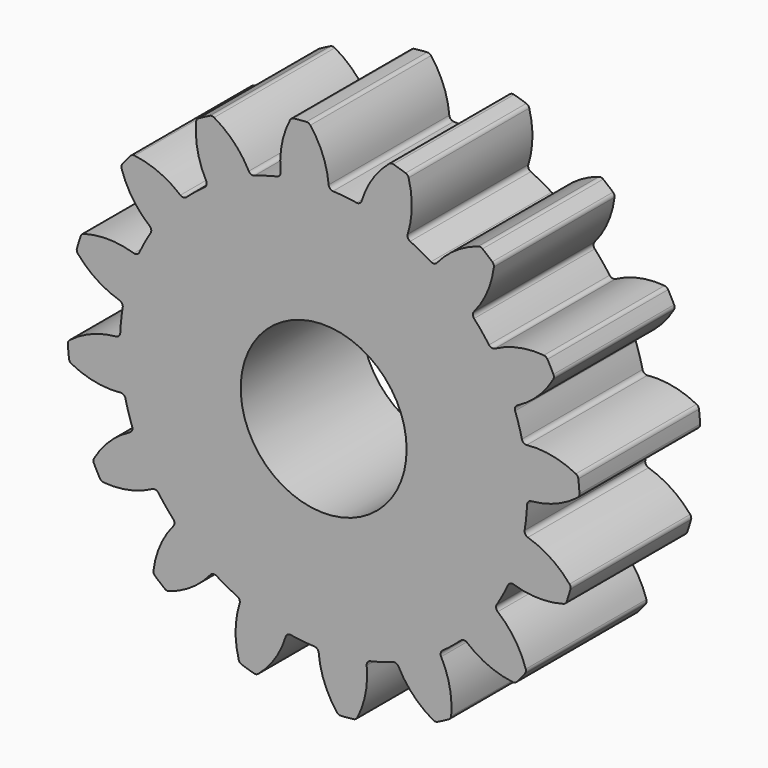
from build123d import *

# Parameters (mm, degrees)
F1_DEPTH = 2
F2_R     = 1.1
F3_DEPTH = 2.001


# Not quite as in the source:
# - a feature names something its author has since deleted; it is built from what else it names


with BuildPart() as f1:
    # F0 (on Front) → F1 (new body)
    with BuildSketch(Plane.XZ):
        with BuildLine():
            ThreePointArc((0.0658501888, 2.7527937353), (-0.0107962206, 3.0784970655), (-0.1768571825, 3.3689812963))
            ThreePointArc((-0.1768571825, 3.3689812963), (-0.2000460149, 3.3871150499), (-0.2290271151, 3.3922774917))
            ThreePointArc((-0.2290271151, 3.3922774917), (-0.3137124222, 3.3854961994), (-0.3982018601, 3.376601143))
            ThreePointArc((-0.3982018601, 3.376601143), (-0.4257409058, 3.3662013384), (-0.4452028358, 3.3441154096))
            ThreePointArc((-0.4452028358, 3.3441154096), (-0.5550599569, 3.0280636032), (-0.5705534857, 2.6938222503))
            ThreePointArc((-0.5705534857, 2.6938222503), (-0.5816569835, 2.6523658625), (-0.6173153418, 2.6284827884))
            ThreePointArc((-0.6173153418, 2.6284827884), (-0.7688345847, 2.5882220502), (-0.9177616204, 2.539234847))
            ThreePointArc((-0.9177616204, 2.539234847), (-1.258998717, 2.3884979026), (-1.5762018248, 2.1921650959))
            ThreePointArc((-1.5762018248, 2.1921650959), (-1.7007802346, 2.09698512), (-1.8196242836, 1.9947349364))
            ThreePointArc((-1.8196242836, 1.9947349364), (-2.0772017217, 1.7248863753), (-2.2951258682, 1.4221101396))
            ThreePointArc((-2.2951258682, 1.4221101396), (-2.3737975114, 1.2865012145), (-2.4444656446, 1.1465547141))
            ThreePointArc((-2.4444656446, 1.1465547141), (-2.5791695941, 0.7986765335), (-2.6646378036, 0.435551806))
            ThreePointArc((-2.6646378036, 0.435551806), (-2.6854256356, 0.2801591612), (-2.6971592704, 0.12382193))
            ThreePointArc((-2.6971592704, 0.12382193), (-2.688482276, -0.2491245706), (-2.6284827884, -0.6173153418))
            ThreePointArc((-2.6284827884, -0.6173153418), (-2.5882220502, -0.7688345847), (-2.539234847, -0.9177616204))
            ThreePointArc((-2.539234847, -0.9177616204), (-2.3884979026, -1.258998717), (-2.1921650959, -1.5762018248))
            ThreePointArc((-2.1921650959, -1.5762018248), (-2.09698512, -1.7007802346), (-1.9947349364, -1.8196242836))
            ThreePointArc((-1.9947349364, -1.8196242836), (-1.7248863753, -2.0772017217), (-1.4221101396, -2.2951258682))
            ThreePointArc((-1.4221101396, -2.2951258682), (-1.2865012145, -2.3737975114), (-1.1465547141, -2.4444656446))
            ThreePointArc((-1.1465547141, -2.4444656446), (-0.7986765335, -2.5791695941), (-0.435551806, -2.6646378036))
            ThreePointArc((-0.435551806, -2.6646378036), (-0.2801591612, -2.6854256356), (-0.12382193, -2.6971592704))
            ThreePointArc((-0.12382193, -2.6971592704), (0.2491245706, -2.688482276), (0.6173153418, -2.6284827884))
            ThreePointArc((0.6173153418, -2.6284827884), (0.7688345847, -2.5882220502), (0.9177616204, -2.539234847))
            ThreePointArc((0.9177616204, -2.539234847), (1.258998717, -2.3884979026), (1.5762018248, -2.1921650959))
            ThreePointArc((1.5762018248, -2.1921650959), (1.7007802346, -2.09698512), (1.8196242836, -1.9947349364))
            ThreePointArc((1.8196242836, -1.9947349364), (2.0772017217, -1.7248863753), (2.2951258682, -1.4221101396))
            ThreePointArc((2.2951258682, -1.4221101396), (2.3737975114, -1.2865012145), (2.4444656446, -1.1465547141))
            ThreePointArc((2.4444656446, -1.1465547141), (2.5791695941, -0.7986765335), (2.6646378036, -0.435551806))
            ThreePointArc((2.6646378036, -0.435551806), (2.6854256356, -0.2801591612), (2.6971592704, -0.12382193))
            ThreePointArc((2.6971592704, -0.12382193), (2.688482276, 0.2491245706), (2.6284827884, 0.6173153418))
            ThreePointArc((2.6284827884, 0.6173153418), (2.5882220502, 0.7688345847), (2.539234847, 0.9177616204))
            ThreePointArc((2.539234847, 0.9177616204), (2.3884979026, 1.258998717), (2.1921650959, 1.5762018248))
            ThreePointArc((2.1921650959, 1.5762018248), (2.09698512, 1.7007802346), (1.9947349364, 1.8196242836))
            ThreePointArc((1.9947349364, 1.8196242836), (1.7248863753, 2.0772017217), (1.4221101396, 2.2951258682))
            ThreePointArc((1.4221101396, 2.2951258682), (1.2865012145, 2.3737975114), (1.1465547141, 2.4444656446))
            ThreePointArc((1.1465547141, 2.4444656446), (0.7986765335, 2.5791695941), (0.435551806, 2.6646378036))
            ThreePointArc((0.435551806, 2.6646378036), (0.2801591612, 2.6854256356), (0.12382193, 2.6971592704))
            ThreePointArc((0.12382193, 2.6971592704), (0.0843822197, 2.7140834836), (0.0658501888, 2.7527937353))
        make_face()
        with BuildLine():
            ThreePointArc((-1.5762018248, 2.1921650959), (-1.258998717, 2.3884979026), (-0.9177616204, 2.539234847))
            ThreePointArc((-0.9177616204, 2.539234847), (-0.9606757776, 2.5397778575), (-0.9926109136, 2.5684495655))
            ThreePointArc((-0.9926109136, 2.5684495655), (-1.1880642308, 2.8400288949), (-1.4526480571, 3.0448525514))
            ThreePointArc((-1.4526480571, 3.0448525514), (-1.4810112319, 3.0527319733), (-1.5097618581, 3.0464108606))
            ThreePointArc((-1.5097618581, 3.0464108606), (-1.5854057918, 3.0077380995), (-1.6600598635, 2.9671874308))
            ThreePointArc((-1.6600598635, 2.9671874308), (-1.6815227913, 2.9470405277), (-1.691051351, 2.9191880319))
            ThreePointArc((-1.691051351, 2.9191880319), (-1.6715983066, 2.5851537366), (-1.5580038326, 2.270425875))
            ThreePointArc((-1.5580038326, 2.270425875), (-1.5523974541, 2.2278760422), (-1.5762018248, 2.1921650959))
        make_face()
        with BuildLine():
            ThreePointArc((-2.2951258682, 1.4221101396), (-2.0772017217, 1.7248863753), (-1.8196242836, 1.9947349364))
            ThreePointArc((-1.8196242836, 1.9947349364), (-1.8594795962, 1.9788140757), (-1.8999560024, 1.9930822324))
            ThreePointArc((-1.8999560024, 1.9930822324), (-2.1844602317, 2.1691920701), (-2.5072864333, 2.2571726072))
            ThreePointArc((-2.5072864333, 2.2571726072), (-2.5365059142, 2.2535981268), (-2.5606490442, 2.2367557919))
            ThreePointArc((-2.5606490442, 2.2367557919), (-2.6157355013, 2.1720791392), (-2.6691888011, 2.10604633))
            ThreePointArc((-2.6691888011, 2.10604633), (-2.6813080748, 2.0792195117), (-2.6794526274, 2.049840739))
            ThreePointArc((-2.6794526274, 2.049840739), (-2.5336509672, 1.7486776481), (-2.3082622193, 1.5013777417))
            ThreePointArc((-2.3082622193, 1.5013777417), (-2.2867994849, 1.4642122902), (-2.2951258682, 1.4221101396))
        make_face()
        with BuildLine():
            ThreePointArc((-2.6646378036, 0.435551806), (-2.5791695941, 0.7986765335), (-2.4444656446, 1.1465547141))
            ThreePointArc((-2.4444656446, 1.1465547141), (-2.4751945026, 1.1165937889), (-2.518050013, 1.1142861968))
            ThreePointArc((-2.518050013, 1.1142861968), (-2.8482919645, 1.1681154163), (-3.1802131787, 1.1258585949))
            ThreePointArc((-3.1802131787, 1.1258585949), (-3.2058405645, 1.1113743944), (-3.2217006257, 1.08657493))
            ThreePointArc((-3.2217006257, 1.08657493), (-3.2478431925, 1.0057408199), (-3.27195794, 0.9242787667))
            ThreePointArc((-3.27195794, 0.9242787667), (-3.27288851, 0.8948561732), (-3.2599315306, 0.8684237753))
            ThreePointArc((-3.2599315306, 0.8684237753), (-3.0099782356, 0.6459812395), (-2.7071086075, 0.5037584573))
            ThreePointArc((-2.7071086075, 0.5037584573), (-2.673057024, 0.4776354902), (-2.6646378036, 0.435551806))
        make_face()
        with BuildLine():
            ThreePointArc((-2.6284827884, -0.6173153418), (-2.688482276, -0.2491245706), (-2.6971592704, 0.12382193))
            ThreePointArc((-2.6971592704, 0.12382193), (-2.7140834836, 0.0843822197), (-2.7527937353, 0.0658501888))
            ThreePointArc((-2.7527937353, 0.0658501888), (-3.0784970655, -0.0107962206), (-3.3689812963, -0.1768571825))
            ThreePointArc((-3.3689812963, -0.1768571825), (-3.3871150499, -0.2000460149), (-3.3922774917, -0.2290271151))
            ThreePointArc((-3.3922774917, -0.2290271151), (-3.3854961994, -0.3137124222), (-3.376601143, -0.3982018601))
            ThreePointArc((-3.376601143, -0.3982018601), (-3.3662013384, -0.4257409058), (-3.3441154096, -0.4452028358))
            ThreePointArc((-3.3441154096, -0.4452028358), (-3.0280636032, -0.5550599569), (-2.6938222503, -0.5705534857))
            ThreePointArc((-2.6938222503, -0.5705534857), (-2.6523658625, -0.5816569835), (-2.6284827884, -0.6173153418))
        make_face()
        with BuildLine():
            ThreePointArc((0.5037584573, 2.7071086075), (0.4776354902, 2.673057024), (0.435551806, 2.6646378036))
            ThreePointArc((0.435551806, 2.6646378036), (0.7986765335, 2.5791695941), (1.1465547141, 2.4444656446))
            ThreePointArc((1.1465547141, 2.4444656446), (1.1165937889, 2.4751945026), (1.1142861968, 2.518050013))
            ThreePointArc((1.1142861968, 2.518050013), (1.1681154163, 2.8482919645), (1.1258585949, 3.1802131787))
            ThreePointArc((1.1258585949, 3.1802131787), (1.1113743944, 3.2058405645), (1.08657493, 3.2217006257))
            ThreePointArc((1.08657493, 3.2217006257), (1.0057408199, 3.2478431925), (0.9242787667, 3.27195794))
            ThreePointArc((0.9242787667, 3.27195794), (0.8948561732, 3.27288851), (0.8684237753, 3.2599315306))
            ThreePointArc((0.8684237753, 3.2599315306), (0.6459812395, 3.0099782356), (0.5037584573, 2.7071086075))
        make_face()
        with BuildLine():
            ThreePointArc((1.5013777417, 2.3082622193), (1.4642122902, 2.2867994849), (1.4221101396, 2.2951258682))
            ThreePointArc((1.4221101396, 2.2951258682), (1.7248863753, 2.0772017217), (1.9947349364, 1.8196242836))
            ThreePointArc((1.9947349364, 1.8196242836), (1.9788140757, 1.8594795962), (1.9930822324, 1.8999560024))
            ThreePointArc((1.9930822324, 1.8999560024), (2.1691920701, 2.1844602317), (2.2571726072, 2.5072864333))
            ThreePointArc((2.2571726072, 2.5072864333), (2.2535981268, 2.5365059142), (2.2367557919, 2.5606490442))
            ThreePointArc((2.2367557919, 2.5606490442), (2.1720791392, 2.6157355013), (2.10604633, 2.6691888011))
            ThreePointArc((2.10604633, 2.6691888011), (2.0792195117, 2.6813080748), (2.049840739, 2.6794526274))
            ThreePointArc((2.049840739, 2.6794526274), (1.7486776481, 2.5336509672), (1.5013777417, 2.3082622193))
        make_face()
        with BuildLine():
            ThreePointArc((2.270425875, 1.5580038326), (2.2278760422, 1.5523974541), (2.1921650959, 1.5762018248))
            ThreePointArc((2.1921650959, 1.5762018248), (2.3884979026, 1.258998717), (2.539234847, 0.9177616204))
            ThreePointArc((2.539234847, 0.9177616204), (2.5397778575, 0.9606757776), (2.5684495655, 0.9926109136))
            ThreePointArc((2.5684495655, 0.9926109136), (2.8400288949, 1.1880642308), (3.0448525514, 1.4526480571))
            ThreePointArc((3.0448525514, 1.4526480571), (3.0527319733, 1.4810112319), (3.0464108606, 1.5097618581))
            ThreePointArc((3.0464108606, 1.5097618581), (3.0077380995, 1.5854057918), (2.9671874308, 1.6600598635))
            ThreePointArc((2.9671874308, 1.6600598635), (2.9470405277, 1.6815227913), (2.9191880319, 1.691051351))
            ThreePointArc((2.9191880319, 1.691051351), (2.5851537366, 1.6715983066), (2.270425875, 1.5580038326))
        make_face()
        with BuildLine():
            ThreePointArc((2.6938222503, 0.5705534857), (2.6523658625, 0.5816569835), (2.6284827884, 0.6173153418))
            ThreePointArc((2.6284827884, 0.6173153418), (2.688482276, 0.2491245706), (2.6971592704, -0.12382193))
            ThreePointArc((2.6971592704, -0.12382193), (2.7140834836, -0.0843822197), (2.7527937353, -0.0658501888))
            ThreePointArc((2.7527937353, -0.0658501888), (3.0784970655, 0.0107962206), (3.3689812963, 0.1768571825))
            ThreePointArc((3.3689812963, 0.1768571825), (3.3871150499, 0.2000460149), (3.3922774917, 0.2290271151))
            ThreePointArc((3.3922774917, 0.2290271151), (3.3854961994, 0.3137124222), (3.376601143, 0.3982018601))
            ThreePointArc((3.376601143, 0.3982018601), (3.3662013384, 0.4257409058), (3.3441154096, 0.4452028358))
            ThreePointArc((3.3441154096, 0.4452028358), (3.0280636032, 0.5550599569), (2.6938222503, 0.5705534857))
        make_face()
        with BuildLine():
            ThreePointArc((2.7071086075, -0.5037584573), (2.673057024, -0.4776354902), (2.6646378036, -0.435551806))
            ThreePointArc((2.6646378036, -0.435551806), (2.5791695941, -0.7986765335), (2.4444656446, -1.1465547141))
            ThreePointArc((2.4444656446, -1.1465547141), (2.4751945026, -1.1165937889), (2.518050013, -1.1142861968))
            ThreePointArc((2.518050013, -1.1142861968), (2.8482919645, -1.1681154163), (3.1802131787, -1.1258585949))
            ThreePointArc((3.1802131787, -1.1258585949), (3.2058405645, -1.1113743944), (3.2217006257, -1.08657493))
            ThreePointArc((3.2217006257, -1.08657493), (3.2478431925, -1.0057408199), (3.27195794, -0.9242787667))
            ThreePointArc((3.27195794, -0.9242787667), (3.27288851, -0.8948561732), (3.2599315306, -0.8684237753))
            ThreePointArc((3.2599315306, -0.8684237753), (3.0099782356, -0.6459812395), (2.7071086075, -0.5037584573))
        make_face()
        with BuildLine():
            ThreePointArc((2.3082622193, -1.5013777417), (2.2867994849, -1.4642122902), (2.2951258682, -1.4221101396))
            ThreePointArc((2.2951258682, -1.4221101396), (2.0772017217, -1.7248863753), (1.8196242836, -1.9947349364))
            ThreePointArc((1.8196242836, -1.9947349364), (1.8594795962, -1.9788140757), (1.8999560024, -1.9930822324))
            ThreePointArc((1.8999560024, -1.9930822324), (2.1844602317, -2.1691920701), (2.5072864333, -2.2571726072))
            ThreePointArc((2.5072864333, -2.2571726072), (2.5365059142, -2.2535981268), (2.5606490442, -2.2367557919))
            ThreePointArc((2.5606490442, -2.2367557919), (2.6157355013, -2.1720791392), (2.6691888011, -2.10604633))
            ThreePointArc((2.6691888011, -2.10604633), (2.6813080748, -2.0792195117), (2.6794526274, -2.049840739))
            ThreePointArc((2.6794526274, -2.049840739), (2.5336509672, -1.7486776481), (2.3082622193, -1.5013777417))
        make_face()
        with BuildLine():
            ThreePointArc((1.5580038326, -2.270425875), (1.5523974541, -2.2278760422), (1.5762018248, -2.1921650959))
            ThreePointArc((1.5762018248, -2.1921650959), (1.258998717, -2.3884979026), (0.9177616204, -2.539234847))
            ThreePointArc((0.9177616204, -2.539234847), (0.9606757776, -2.5397778575), (0.9926109136, -2.5684495655))
            ThreePointArc((0.9926109136, -2.5684495655), (1.1880642308, -2.8400288949), (1.4526480571, -3.0448525514))
            ThreePointArc((1.4526480571, -3.0448525514), (1.4810112319, -3.0527319733), (1.5097618581, -3.0464108606))
            ThreePointArc((1.5097618581, -3.0464108606), (1.5854057918, -3.0077380995), (1.6600598635, -2.9671874308))
            ThreePointArc((1.6600598635, -2.9671874308), (1.6815227913, -2.9470405277), (1.691051351, -2.9191880319))
            ThreePointArc((1.691051351, -2.9191880319), (1.6715983066, -2.5851537366), (1.5580038326, -2.270425875))
        make_face()
        with BuildLine():
            ThreePointArc((0.5705534857, -2.6938222503), (0.5816569835, -2.6523658625), (0.6173153418, -2.6284827884))
            ThreePointArc((0.6173153418, -2.6284827884), (0.2491245706, -2.688482276), (-0.12382193, -2.6971592704))
            ThreePointArc((-0.12382193, -2.6971592704), (-0.0843822197, -2.7140834836), (-0.0658501888, -2.7527937353))
            ThreePointArc((-0.0658501888, -2.7527937353), (0.0107962206, -3.0784970655), (0.1768571825, -3.3689812963))
            ThreePointArc((0.1768571825, -3.3689812963), (0.2000460149, -3.3871150499), (0.2290271151, -3.3922774917))
            ThreePointArc((0.2290271151, -3.3922774917), (0.3137124222, -3.3854961994), (0.3982018601, -3.376601143))
            ThreePointArc((0.3982018601, -3.376601143), (0.4257409058, -3.3662013384), (0.4452028358, -3.3441154096))
            ThreePointArc((0.4452028358, -3.3441154096), (0.5550599569, -3.0280636032), (0.5705534857, -2.6938222503))
        make_face()
        with BuildLine():
            ThreePointArc((-0.435551806, -2.6646378036), (-0.7986765335, -2.5791695941), (-1.1465547141, -2.4444656446))
            ThreePointArc((-1.1465547141, -2.4444656446), (-1.1165937889, -2.4751945026), (-1.1142861968, -2.518050013))
            ThreePointArc((-1.1142861968, -2.518050013), (-1.1681154163, -2.8482919645), (-1.1258585949, -3.1802131787))
            ThreePointArc((-1.1258585949, -3.1802131787), (-1.1113743944, -3.2058405645), (-1.08657493, -3.2217006257))
            ThreePointArc((-1.08657493, -3.2217006257), (-1.0057408199, -3.2478431925), (-0.9242787667, -3.27195794))
            ThreePointArc((-0.9242787667, -3.27195794), (-0.8948561732, -3.27288851), (-0.8684237753, -3.2599315306))
            ThreePointArc((-0.8684237753, -3.2599315306), (-0.6459812395, -3.0099782356), (-0.5037584573, -2.7071086075))
            ThreePointArc((-0.5037584573, -2.7071086075), (-0.4776354902, -2.673057024), (-0.435551806, -2.6646378036))
        make_face()
        with BuildLine():
            ThreePointArc((-1.4221101396, -2.2951258682), (-1.7248863753, -2.0772017217), (-1.9947349364, -1.8196242836))
            ThreePointArc((-1.9947349364, -1.8196242836), (-1.9788140757, -1.8594795962), (-1.9930822324, -1.8999560024))
            ThreePointArc((-1.9930822324, -1.8999560024), (-2.1691920701, -2.1844602317), (-2.2571726072, -2.5072864333))
            ThreePointArc((-2.2571726072, -2.5072864333), (-2.2535981268, -2.5365059142), (-2.2367557919, -2.5606490442))
            ThreePointArc((-2.2367557919, -2.5606490442), (-2.1720791392, -2.6157355013), (-2.10604633, -2.6691888011))
            ThreePointArc((-2.10604633, -2.6691888011), (-2.0792195117, -2.6813080748), (-2.049840739, -2.6794526274))
            ThreePointArc((-2.049840739, -2.6794526274), (-1.7486776481, -2.5336509672), (-1.5013777417, -2.3082622193))
            ThreePointArc((-1.5013777417, -2.3082622193), (-1.4642122902, -2.2867994849), (-1.4221101396, -2.2951258682))
        make_face()
        with BuildLine():
            ThreePointArc((-2.1921650959, -1.5762018248), (-2.3884979026, -1.258998717), (-2.539234847, -0.9177616204))
            ThreePointArc((-2.539234847, -0.9177616204), (-2.5397778575, -0.9606757776), (-2.5684495655, -0.9926109136))
            ThreePointArc((-2.5684495655, -0.9926109136), (-2.8400288949, -1.1880642308), (-3.0448525514, -1.4526480571))
            ThreePointArc((-3.0448525514, -1.4526480571), (-3.0527319733, -1.4810112319), (-3.0464108606, -1.5097618581))
            ThreePointArc((-3.0464108606, -1.5097618581), (-3.0077380995, -1.5854057918), (-2.9671874308, -1.6600598635))
            ThreePointArc((-2.9671874308, -1.6600598635), (-2.9470405277, -1.6815227913), (-2.9191880319, -1.691051351))
            ThreePointArc((-2.9191880319, -1.691051351), (-2.5851537366, -1.6715983066), (-2.270425875, -1.5580038326))
            ThreePointArc((-2.270425875, -1.5580038326), (-2.2278760422, -1.5523974541), (-2.1921650959, -1.5762018248))
        make_face()
    extrude(amount=F1_DEPTH)

    # F2 (on face) → F3 (cut, through all)
    with BuildSketch(Plane.XZ.offset(2)):
        Circle(F2_R)
    extrude(amount=-F3_DEPTH, mode=Mode.SUBTRACT)


solid = f1.part
